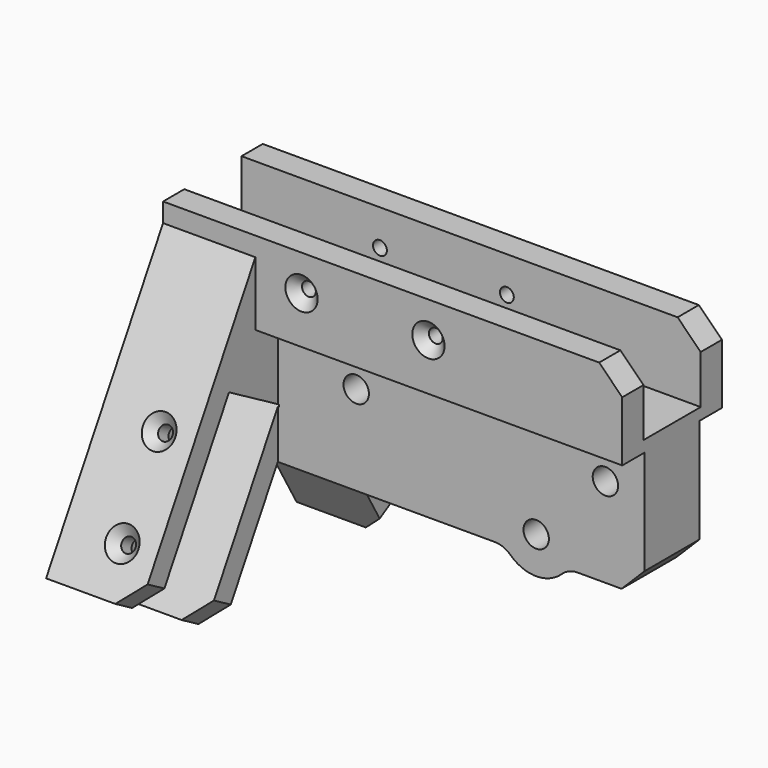
from build123d import *

# Parameters (mm, degrees)
F0_W         = 15
F0_H         = 15
F1_DEPTH     = 20
F3_DEPTH     = 15
F4_R         = 1.5
F5_DEPTH     = 5.5
F6_R         = 1.5
F7_DEPTH     = 5.5
F8_W         = 15
F8_H         = 15
F9_DEPTH     = 47.5
F10_R        = 4
F11_DEPTH    = 19.374355653
F13_DEPTH    = 47.5
F14_R        = 2.75
F15_DEPTH    = 52.6205461814
F16_DEPTH    = 20
F17_W        = 67.5
F17_H        = 14.8660254038
F17_R        = 4
F18_DEPTH    = 11
F19_W        = 14.8660254038
F19_H        = 26.3910161514
F20_DEPTH    = 67.501
F21_SIZE     = 5
F22_R        = 1.5
F23_DEPTH    = 58.6875334795
F24_W        = 15.5
F24_H        = 15.5
F25_DEPTH    = 67.501
F26_W        = 15.5
F26_H        = 15.5
F27_DEPTH    = 51.2593302492
F28_W        = 15.5
F28_H        = 15.5
F29_DEPTH    = 51.2593302492
F30_DEPTH    = 32
F31_R        = 2.75
F32_DEPTH    = 52.6205461814
F33_R        = 8
F33_R_2      = 2.75
F34_DEPTH    = 14.8660254038
F36_DEPTH    = 99.5
F37_W        = 27
F37_H        = 4.75
F38_DEPTH    = 99.501
F39_T1_DEPTH = 40.5828552834
F39_T3_DEPTH = 31.4668298797
F39_T5_DEPTH = 31.4668298797
F40_R        = 5
F41_SIZE     = 2


# Not quite as in the source:
# - a fillet or chamfer that OpenCascade refuses, or shapes differently, is made with other operations: its cross-section is extruded or revolved along the edge and cut away or added
# - an extrude ends at something that could not be found from the text; its depth is read off the source's solid


with BuildPart() as f1:
    # F0 (on Right) → F1 (new body)
    with BuildSketch(Plane.YZ):
        Polygon((45.1865334795, -51.2653718044), (8.3715789032, 12.5), (-8.3715789032, 12.5), (-45.1865334795, -51.2653718044), (-22.6698729811, -64.2653718044), (0, -25), (22.6698729811, -64.2653718044), align=None)
        Rectangle(F0_W, F0_H, mode=Mode.SUBTRACT)
    extrude(amount=F1_DEPTH)

    # F2 (on face) → F3 (cut)
    with BuildSketch(Plane.YZ.offset(20)):
        Polygon((-20.4233937587, -19.374355653), (-40.4233937587, -54.0153718044), (-27.4330127019, -61.5153718044), (-7.4330127019, -26.874355653), align=None)
        Polygon((27.4330127019, -61.5153718044), (40.4233937587, -54.0153718044), (20.4233937587, -19.374355653), (7.4330127019, -26.874355653), align=None)
    extrude(amount=-F3_DEPTH, mode=Mode.SUBTRACT)

    # F4 (on face) → F5 (cut, through all)
    with BuildSketch(Plane(origin=(0, -11.6913429511, 6.75), x_dir=(1, 0, 0), z_dir=(0, -0.8660254038, 0.5))):
        with Locations((12.5, -36.9903810568)):
            Circle(F4_R)
        with Locations((12.5, -56.9903810568)):
            Circle(F4_R)
    extrude(amount=-F5_DEPTH, mode=Mode.SUBTRACT)

    # F6 (on face) → F7 (cut, through all)
    with BuildSketch(Plane(origin=(0, 11.6913429511, 6.75), x_dir=(-1, 0, 0), z_dir=(0, 0.8660254038, 0.5))):
        with Locations((-12.5, -56.9903810568)):
            Circle(F6_R)
        with Locations((-12.5, -36.9903810568)):
            Circle(F6_R)
    extrude(amount=-F7_DEPTH, mode=Mode.SUBTRACT)

    # F8 (on face) → F9 (join)
    with BuildSketch(Plane.YZ.offset(20)):
        Polygon((8.3715789032, 12.5), (-8.3715789032, 12.5), (-13.5, 3.6173140978), (-13.5, -23.3715789032), (-7.4330127019, -26.874355653), (7.4330127019, -26.874355653), (13.5, -23.3715789032), (13.5, 3.6173140978), align=None)
        Rectangle(F8_W, F8_H, mode=Mode.SUBTRACT)
    extrude(amount=F9_DEPTH)

    # F10 (on face) → F11 (cut, through all)
    with BuildSketch(Plane(origin=(0, 0, -26.874355653), x_dir=(1, 0, 0), z_dir=(0, 0, -1))):
        with Locations((50, 0)):
            Circle(F10_R)
    extrude(amount=-F11_DEPTH, mode=Mode.SUBTRACT)

    # F12 (on face) → F13 (cut, through all)
    with BuildSketch(Plane.YZ.offset(67.5)):
        Polygon((-13.5, -23.3715789032), (-7.4330127019, -26.874355653), (-7.4330127019, -10.25), (-13.5, -10.25), align=None)
        Polygon((7.4330127019, -10.25), (7.4330127019, -26.874355653), (13.5, -23.3715789032), (13.5, -10.25), align=None)
    extrude(amount=-F13_DEPTH, mode=Mode.SUBTRACT)

    # F14 (on face) → F15 (cut, through all)
    with BuildSketch(Plane.XZ.offset(7.4330127019)):
        with Locations((36.9997965198, -18.5)):
            Circle(F14_R)
    extrude(amount=-F15_DEPTH, mode=Mode.SUBTRACT)

    # F16 (add, through all): a face of the model
    f16_faces = [f1.faces().sort_by_distance(p)[0] for p in [
        (20, 0, -26.2495704353),
    ]]
    extrude(f16_faces, amount=F16_DEPTH)

    # F17 (on face) → F18 (join, through all)
    with BuildSketch(Plane(origin=(0, 0, -26.874355653), x_dir=(1, 0, 0), z_dir=(0, 0, -1))):
        with Locations((33.75, 0)):
            Rectangle(F17_W, F17_H)
        with Locations((50, 0)):
            Circle(F17_R, mode=Mode.SUBTRACT)
    extrude(amount=F18_DEPTH)

    # F19 (on face) → F20 (cut, through all)
    with BuildSketch(Plane(origin=(0, 0, 0), x_dir=(0, -1, 0), z_dir=(-1, 0, 0))):
        with Locations((0, -51.0698637287)):
            Rectangle(F19_W, F19_H)
    extrude(amount=-F20_DEPTH, mode=Mode.SUBTRACT)

    # F21
    f21_edges = [f1.edges().sort_by_distance(p)[0] for p in [
        (20, -42.804964, -52.640372),
        (20, -25.051443, -62.890372),
        (20, 25.051443, -62.890372),
        (20, 42.804964, -52.640372),
    ]]
    chamfer(f21_edges, length=F21_SIZE)

    # F22 (on face) → F23 (cut, through all)
    with BuildSketch(Plane.XZ.offset(13.5)):
        with Locations((30, 0)):
            Circle(F22_R)
        with Locations((57.5, 0)):
            Circle(F22_R)
    extrude(amount=-F23_DEPTH, mode=Mode.SUBTRACT)

    # F24 (on face) → F25 (cut, through all)
    with BuildSketch(Plane(origin=(0, 0, 0), x_dir=(0, -1, 0), z_dir=(-1, 0, 0))):
        Rectangle(F24_W, F24_H)
    extrude(amount=-F25_DEPTH, mode=Mode.SUBTRACT)

    # F26 (on face) → F27 (cut, through all)
    with BuildSketch(Plane(origin=(0, -13.4951905284, -23.374355653), x_dir=(1, 0, 0), z_dir=(0, -0.5, -0.8660254038))):
        with Locations((12.5, 0.5)):
            Rectangle(F26_W, F26_H)
    extrude(amount=F27_DEPTH, mode=Mode.SUBTRACT)

    # F28 (on face) → F29 (cut, through all)
    with BuildSketch(Plane(origin=(0, 13.4951905284, -23.374355653), x_dir=(1, 0, 0), z_dir=(0, 0.5, -0.8660254038))):
        with Locations((12.5, -0.5)):
            Rectangle(F28_W, F28_H)
    extrude(amount=F29_DEPTH, mode=Mode.SUBTRACT)

    # F30 (add): a face of the model
    f30_faces = [f1.faces().sort_by_distance(p)[0] for p in [
        (67.5, 0, -13.0224065519),
    ]]
    extrude(f30_faces, amount=F30_DEPTH)

    # F31 (on face) → F32 (cut, through all)
    with BuildSketch(Plane.XZ.offset(7.4330127019)):
        with Locations((91, -18.5)):
            Circle(F31_R)
        with Locations((76, -33.5)):
            Circle(F31_R)
    extrude(amount=-F32_DEPTH, mode=Mode.SUBTRACT)

    # F33 (on face) → F34 (join, through all)
    with BuildSketch(Plane.XZ.offset(7.4330127019)):
        with Locations((76, -33.5)):
            Circle(F33_R)
        with Locations((76, -33.5)):
            Circle(F33_R_2, mode=Mode.SUBTRACT)
    extrude(amount=-F34_DEPTH)

    # F35 (on face) → F36 (join, through all)
    with BuildSketch(Plane.YZ.offset(99.5)):
        Polygon((-13.5, 3.6173140978), (-8.3715789032, 12.5), (-13.5, 12.5), align=None)
        Polygon((13.5, 12.5), (8.3715789032, 12.5), (13.5, 3.6173140978), align=None)
    extrude(amount=-F36_DEPTH)

    # F37 (on face) → F38 (cut, through all)
    with BuildSketch(Plane.YZ.offset(99.5)):
        with Locations((0, 10.125)):
            Rectangle(F37_W, F37_H)
    extrude(amount=-F38_DEPTH, mode=Mode.SUBTRACT)

    # F39: chamfer of 5 on 5 edges, made by hand

    # F39_s2 → F39_t1 (cut)
    with BuildSketch(Plane.XZ.offset(-20.2914276417)):
        Polygon((99.5, -32.874355653), (94.5, -37.874355653), (99.5, -37.874355653), align=None)
    extrude(amount=F39_T1_DEPTH, mode=Mode.SUBTRACT)

    # F39_s4 → F39_t3 (cut)
    with BuildSketch(Plane.XZ.offset(-5.1084149398)):
        Polygon((94.5, 7.75), (99.5, 2.75), (99.5, 7.75), align=None)
    extrude(amount=F39_T3_DEPTH, mode=Mode.SUBTRACT)

    # F39_s6 → F39_t5 (cut)
    with BuildSketch(Plane.XZ.offset(-26.3584149398)):
        Polygon((94.5, 7.75), (99.5, 2.75), (99.5, 7.75), align=None)
    extrude(amount=F39_T5_DEPTH, mode=Mode.SUBTRACT)

    # F40
    f40_edges = [f1.edges().sort_by_distance(p)[0] for p in [
        (69.301865, 0, -37.874356),
        (82.698135, 0, -37.874356),
    ]]
    fillet(f40_edges, radius=F40_R)

    # F41
    f41_edges = [f1.edges().sort_by_distance(p)[0] for p in [
        (28.5, -13.5, 0),
        (56, -13.5, 0),
        (11, -30.186533, -25.28461),
        (11, -40.186533, -42.605118),
        (56, 13.5, 0),
        (28.5, 13.5, 0),
        (14, 30.186533, -25.28461),
        (14, 40.186533, -42.605118),
    ]]
    chamfer(f41_edges, length=F41_SIZE)


solid = f1.part
